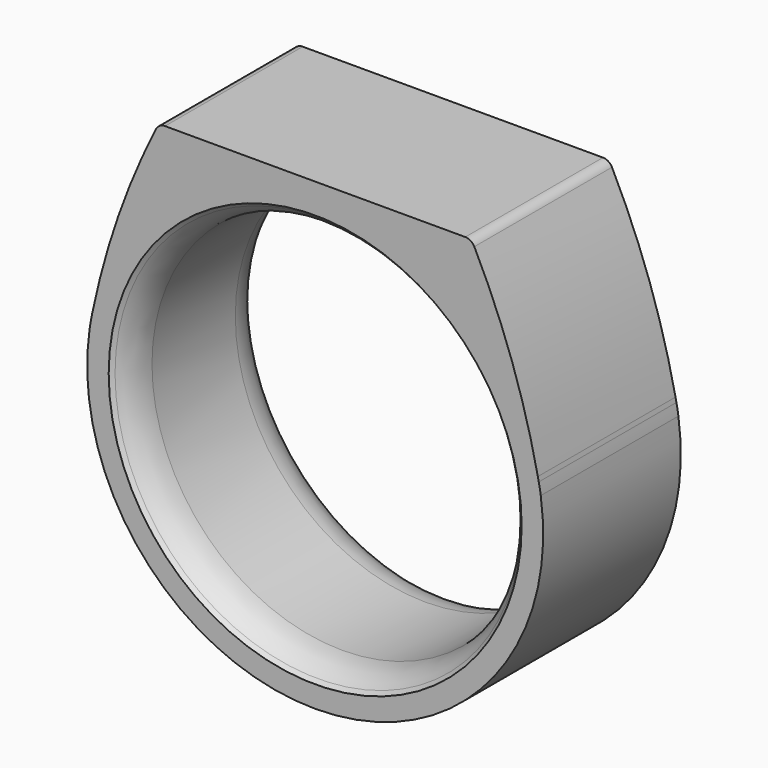
from build123d import *

# Parameters (mm, degrees)
F0_R          = 8.85
F1_DEPTH      = 4
F1_DEPTH_BACK = 4
F2_T1_DEPTH   = 10.0905704575
F3_SIZE       = 0.75
F4_R          = 0.4704417071


# Not quite as in the source:
# - a fillet or chamfer that OpenCascade refuses, or shapes differently, is made with other operations: its cross-section is extruded or revolved along the edge and cut away or added


with BuildPart() as f1:
    # F0 (on Front) → F1 (new body, two sides)
    with BuildSketch(Plane.XZ) as f1_sk:
        with BuildLine():
            ThreePointArc((-10.4187088027, 1.9520519678), (-0.9802261707, -10.55457989), (10.6, 0))
            ThreePointArc((10.6, 0), (10.55457989, 0.9802261707), (10.4187088027, 1.9520519678))
            ThreePointArc((10.4187088027, 1.9520519678), (10.3862442109, 2.1135702761), (10.3530039199, 2.2749307319))
            ThreePointArc((10.3530039199, 2.2749307319), (0, 10.6), (-10.3530039199, 2.2749307319))
            ThreePointArc((-10.3530039199, 2.2749307319), (-10.3862442109, 2.1135702761), (-10.4187088027, 1.9520519678))
        make_face()
        Circle(F0_R, mode=Mode.SUBTRACT)
        with BuildLine():
            ThreePointArc((-10.3530039199, 2.2749307319), (0, 10.6), (10.3530039199, 2.2749307319))
            ThreePointArc((10.3530039199, 2.2749307319), (9.1045987077, 6.7318445783), (7.2673073852, 10.9800156206))
            Line((7.2673073852, 10.9800156206), (0, 10.9800156206))
            Line((0, 10.9800156206), (-7.2673073852, 10.9800156206))
            ThreePointArc((-7.2673073852, 10.9800156206), (-9.1045987077, 6.7318445783), (-10.3530039199, 2.2749307319))
        make_face()
    extrude(amount=F1_DEPTH)
    extrude(f1_sk.sketch, amount=-F1_DEPTH_BACK)

    # F2: fillet of radius 10 on 2 edges, made by hand

    # F2_s2 → F2_t1 (cut)
    with BuildSketch(Plane.XZ.offset(-5.0452852288)):
        with BuildLine():
            ThreePointArc((-10.4875868169, 1.5396502065), (-10.4450837448, 1.8044143565), (-10.3954968357, 2.0679436806))
            ThreePointArc((-10.3954968357, 2.0679436806), (-10.4071527555, 2.010007826), (-10.4187088027, 1.9520519678))
            ThreePointArc((-10.4187088027, 1.9520519678), (-10.4551813918, 1.7461907295), (-10.4875868169, 1.5396502065))
        make_face()
        with BuildLine():
            ThreePointArc((10.4875868169, 1.5396502065), (10.4450837448, 1.8044143565), (10.3954968357, 2.0679436806))
            ThreePointArc((10.3954968357, 2.0679436806), (10.4071527555, 2.010007826), (10.4187088027, 1.9520519678))
            ThreePointArc((10.4187088027, 1.9520519678), (10.4551813918, 1.7461907295), (10.4875868169, 1.5396502065))
        make_face()
    extrude(amount=F2_T1_DEPTH, mode=Mode.SUBTRACT)

    # F3
    f3_edges = [f1.edges().sort_by_distance(p)[0] for p in [
        (-8.85, 4, 0),
        (-8.85, -4, 0),
    ]]
    chamfer(f3_edges, length=F3_SIZE)

    # F4
    f4_edges = [f1.edges().sort_by_distance(p)[0] for p in [
        (-7.267307, 0, 10.980016),
        (7.267307, 0, 10.980016),
    ]]
    fillet(f4_edges, radius=F4_R)

    # F5: fillet of radius 2 on 2 edges, made by hand

    # F5_s1 → F5_t2 (revolve, cut)
    with BuildSketch(Plane.XY):
        with BuildLine():
            add(Edge.make_bspline(
                [(8.85, -2.4215728753), (8.85, -3.25), (9.4357864376, -3.8357864376)],
                knots=[0, 0, 0, 1, 1, 1], degree=2, weights=[1, 1, 1]))
            Line((9.4357864376, -3.8357864376), (8.85, -3.25))
            Line((8.85, -3.25), (8.85, -2.4215728753))
        make_face()
    revolve(axis=Axis((0, -3.25, 0), (0, -1, 0)), mode=Mode.SUBTRACT)

    # F5_s3 → F5_t4 (revolve, cut)
    with BuildSketch(Plane.XY):
        with BuildLine():
            add(Edge.make_bspline(
                [(9.4357864376, 3.8357864376), (8.85, 3.25), (8.85, 2.4215728753)],
                knots=[0, 0, 0, 1, 1, 1], degree=2, weights=[1, 1, 1]))
            Line((8.85, 2.4215728753), (8.85, 3.25))
            Line((8.85, 3.25), (9.4357864376, 3.8357864376))
        make_face()
    revolve(axis=Axis((0, 3.25, 0), (0, -1, 0)), mode=Mode.SUBTRACT)


solid = f1.part
